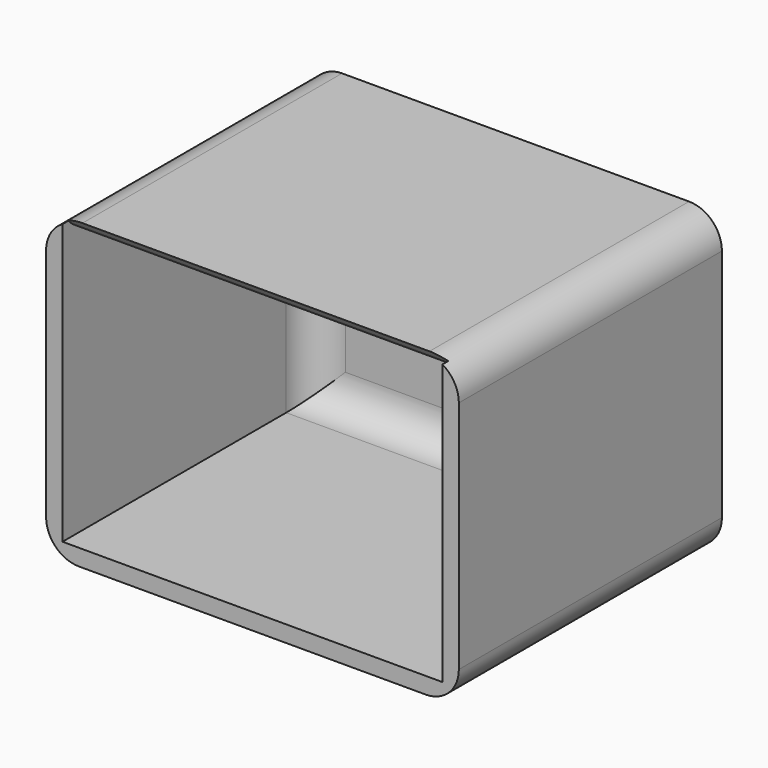
from build123d import *

# Parameters (mm, degrees)
F0_W        = 62.7580881119
F0_H        = 45.6833392382
F1_DEPTH    = 50
F2_T        = -2.5
F3_R        = 5
F4_T1_DEPTH = 40.6833392382
F4_T3_DEPTH = 57.7580881119
F4_T5_DEPTH = 57.7580881119


# Not quite as in the source:
# - a fillet or chamfer that OpenCascade refuses, or shapes differently, is made with other operations: its cross-section is extruded or revolved along the edge and cut away or added


with BuildPart() as f1:
    # F0 (on Front) → F1 (new body)
    with BuildSketch(Plane.XZ):
        with Locations((31.3790440559, 22.8416696191)):
            Rectangle(F0_W, F0_H)
    extrude(amount=-F1_DEPTH)

    # F2
    f2_openings = [f1.faces().sort_by_distance(p)[0] for p in [
        (31.379044, 0, 22.84167),
    ]]
    offset(amount=F2_T, openings=f2_openings)

    # F3
    f3_edges = [f1.edges().sort_by_distance(p)[0] for p in [
        (0, 25, 45.683339),
        (62.758088, 25, 45.683339),
        (62.758088, 25, 0),
        (0, 25, 0),
    ]]
    fillet(f3_edges, radius=F3_R)

    # F4: fillet of radius 5 on 5 edges, made by hand

    # F4_s2 → F4_t1 (join)
    with BuildSketch(Plane.XY.offset(2.5)):
        with BuildLine():
            ThreePointArc((2.5, 42.5), (3.9644660941, 46.0355339059), (7.5, 47.5))
            Line((7.5, 47.5), (2.5, 47.5))
            Line((2.5, 47.5), (2.5, 42.5))
        make_face()
        with BuildLine():
            ThreePointArc((60.2580881119, 42.5), (58.7936220178, 46.0355339059), (55.2580881119, 47.5))
            Line((55.2580881119, 47.5), (60.2580881119, 47.5))
            Line((60.2580881119, 47.5), (60.2580881119, 42.5))
        make_face()
    extrude(amount=F4_T1_DEPTH)

    # F4_s4 → F4_t3 (join)
    with BuildSketch(Plane.YZ.offset(2.5)):
        with BuildLine():
            ThreePointArc((42.5, 2.5), (46.0355339059, 3.9644660941), (47.5, 7.5))
            Line((47.5, 7.5), (47.5, 2.5))
            Line((47.5, 2.5), (42.5, 2.5))
        make_face()
        with BuildLine():
            ThreePointArc((42.5, 43.1833392382), (46.0355339059, 41.7188731441), (47.5, 38.1833392382))
            Line((47.5, 38.1833392382), (47.5, 43.1833392382))
            Line((47.5, 43.1833392382), (42.5, 43.1833392382))
        make_face()
    extrude(amount=F4_T3_DEPTH)

    # F4_s6 → F4_t5 (cut)
    with BuildSketch(Plane.YZ.offset(2.5)):
        with BuildLine():
            ThreePointArc((0, 48.1833392382), (1.4644660941, 44.6478053322), (5, 43.1833392382))
            Line((5, 43.1833392382), (0, 43.1833392382))
            Line((0, 43.1833392382), (0, 48.1833392382))
        make_face()
    extrude(amount=F4_T5_DEPTH, mode=Mode.SUBTRACT)


solid = f1.part
